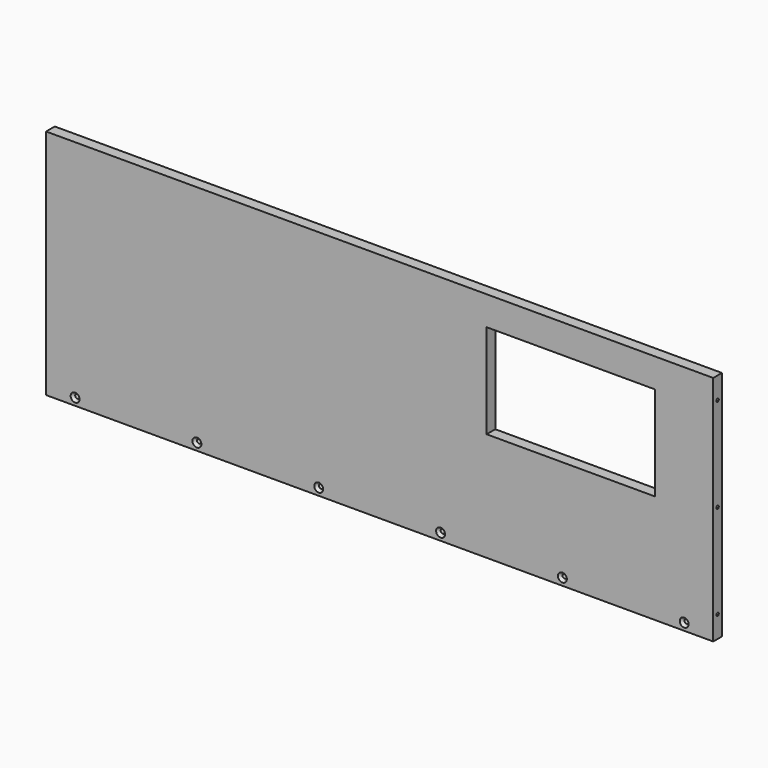
from build123d import *

# Parameters (mm, degrees)
F0_W           = 584.2
F0_H           = 203.2
F1_DEPTH       = 9.525
F3_D           = 3.6576
F3_DEPTH       = 10.3124
F3_CSINK_D     = 7.7978
F3_CSINK_ANGLE = 82
F3_TIP         = 1.0988539001
F4_W           = 147.6502
F4_H           = 82.55
F5_DEPTH       = 9.526
F7_D           = 2.7051
F7_DEPTH       = 13.49375
F7_TIP         = 0.8126940303
F9_D           = 2.7051
F9_DEPTH       = 13.49375
F9_TIP         = 0.8126940303


# Not quite as in the source:
# - a feature names something its author has since deleted; it is built from what else it names


with BuildPart() as f1:
    # F0 (on Front) → F1 (new body)
    with BuildSketch(Plane.XZ):
        with Locations((-292.1, 87.2551402715)):
            Rectangle(F0_W, F0_H)
    extrude(amount=F1_DEPTH)

    # F3
    with Locations(Plane.XZ.offset(9.525)):
        with Locations((-558.8, -7.9948597285), (-345.44, -7.9948597285), (-452.12, -7.9948597285), (-238.76, -7.9948597285), (-132.08, -7.9948597285), (-25.4, -7.9948597285)):
            CounterSinkHole(F3_D / 2, F3_CSINK_D / 2, depth=F3_DEPTH, counter_sink_angle=F3_CSINK_ANGLE)
            with Locations((0, 0, -(F3_DEPTH + F3_TIP / 2))):  # 118° drill point
                Cone(0, F3_D / 2, F3_TIP, mode=Mode.SUBTRACT)

    # F4 (on face) → F5 (cut, through all)
    with BuildSketch(Plane.XZ.offset(9.525)):
        with Locations((-124.6251, 122.1801402715)):
            Rectangle(F4_W, F4_H)
    extrude(amount=-F5_DEPTH, mode=Mode.SUBTRACT)

    # F7
    with Locations(Plane(origin=(-584.2, 0, 0), x_dir=(0, -1, 0), z_dir=(-1, 0, 0))):
        with Locations((4.7625, 169.8051402715), (4.7625, 87.2551402715), (4.7625, 4.7051402715)):
            Hole(F7_D / 2, depth=F7_DEPTH)
            with Locations((0, 0, -(F7_DEPTH + F7_TIP / 2))):  # 118° drill point
                Cone(0, F7_D / 2, F7_TIP, mode=Mode.SUBTRACT)

    # F9
    with Locations(Plane.YZ):
        with Locations((-4.7625, 4.7051402715), (-4.7625, 87.2551402715), (-4.7625, 169.8051402715)):
            Hole(F9_D / 2, depth=F9_DEPTH)
            with Locations((0, 0, -(F9_DEPTH + F9_TIP / 2))):  # 118° drill point
                Cone(0, F9_D / 2, F9_TIP, mode=Mode.SUBTRACT)


solid = f1.part
